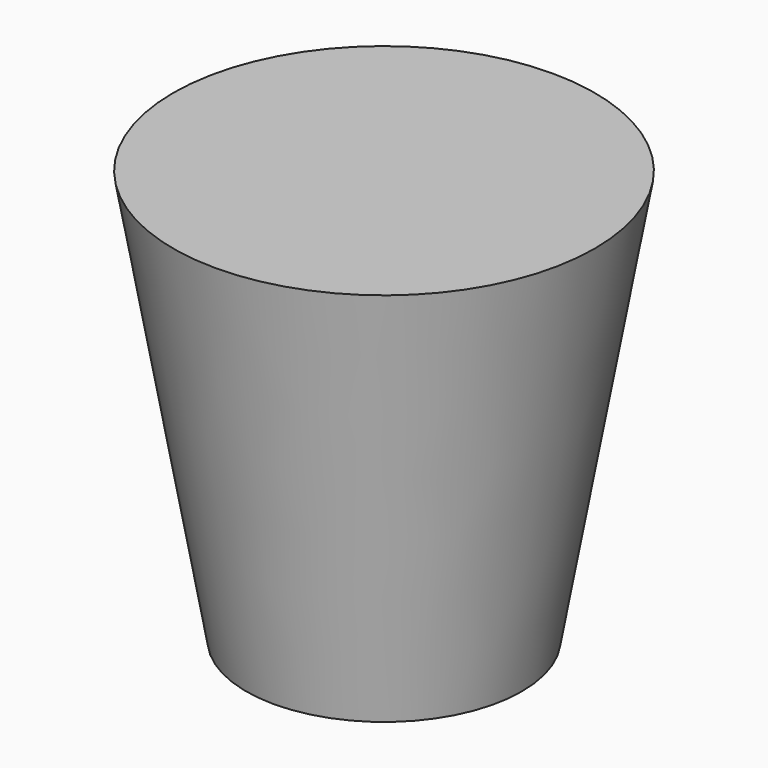
from build123d import *

# Parameters (mm, degrees)
F0_R     = 50
F1_DEPTH = 150
F1_TAPER = -10


with BuildPart() as f1:
    # F0 (on Top) → F1 (new body)
    with BuildSketch(Plane.XY):
        Circle(F0_R)
    extrude(amount=F1_DEPTH, taper=F1_TAPER)


solid = f1.part
